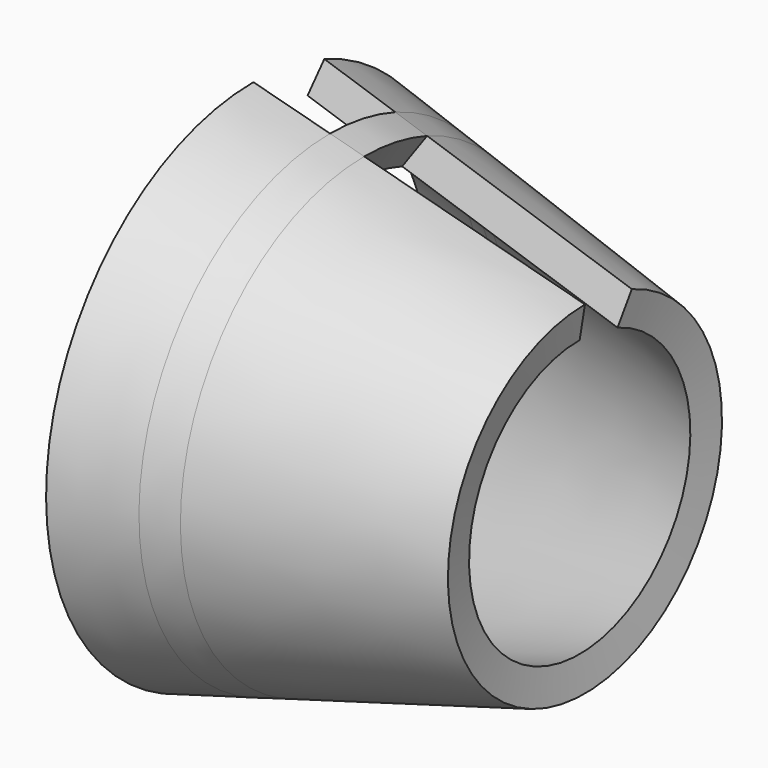
from build123d import *
from build123d import SkipClean  # not in build123d's __all__

# Parameters (mm, degrees)
F1_ANGLE = 340


with BuildPart() as f1:
    # F0 (on Front) → F1 (revolve)
    with BuildSketch(Plane.XZ):
        Polygon((-48.5273150222, 95.1958908392), (-51.4471201788, 83.3390055934), (71.3136761488, 50.8), (73.2494630124, 62.9177093663), align=None)
    revolve(axis=Axis((3.1582843512, 0, 0), (1, 0, 0)), revolution_arc=F1_ANGLE)

    # F2 (on face) → F3 (revolve)
    with BuildSketch(Plane(origin=(0, 0, 0), x_dir=(1, 0, 0), z_dir=(0, -0.9396926208, 0.3420201433))):
        Polygon((-7.8220407683, 84.4065412565), (-20.3833373413, 87.7360414852), (-25.218585377, 76.3868639802), (-13.9751803482, 73.4066843946), align=None)
    with SkipClean():  # cleaning this boolean's faces spoils the solid; the shape is the same uncleaned
        revolve(axis=Axis((73.2494630124, 0, 0), (-1, 0, 0)))


solid = f1.part
